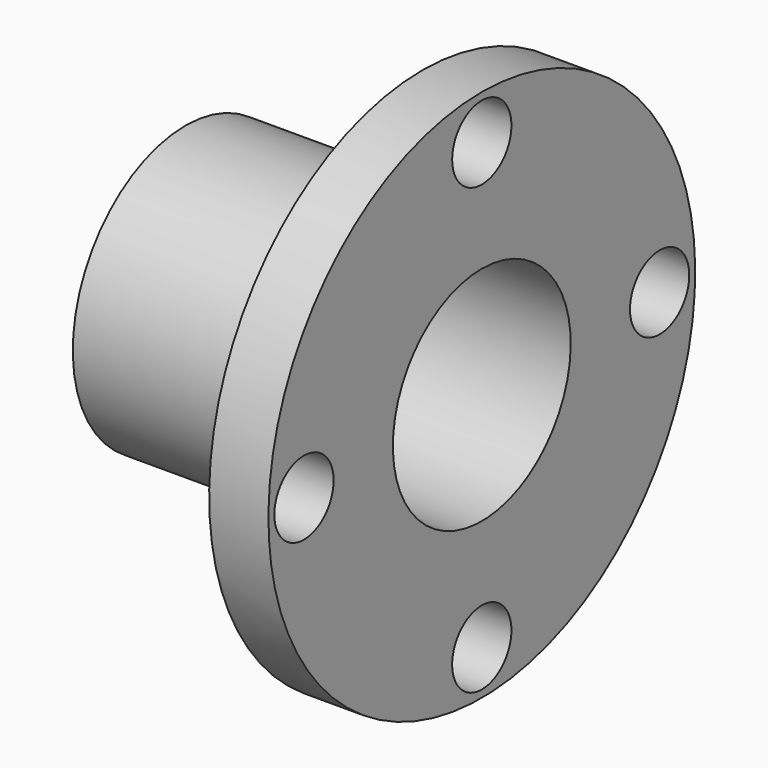
from build123d import *

# Parameters (mm, degrees)
F2_R            = 12.5
F3_DEPTH        = 25
F3_COPIES_COUNT = 4


# Not quite as in the source:
# - a pattern or mirror of a feature is missing from the dataset's text; its kind, count and spacing are read off the source's solid


with BuildPart() as f1:
    # F0 (on Front) → F1 (revolve)
    with BuildSketch(Plane.XZ):
        Polygon((-100, 37.5), (0, 37.5), (0, 90), (-20, 90), (-20, 47.5), (-100, 47.5), align=None)
    revolve(axis=Axis((-58.4905732034, 0, 0), (-1, 0, 0)))

    # F2 (on face) → F3 (cut)
    with BuildSketch(Plane(origin=(-20, 0, 0), x_dir=(0, -1, 0), z_dir=(-1, 0, 0))):
        with Locations((0, 75)):
            Circle(F2_R)
    f3 = extrude(amount=-F3_DEPTH, mode=Mode.SUBTRACT)

    # F3_copies: F3 ×4 about axis
    f3_copies_axis = Axis((0, 0, 0), (1, 0, 0))
    for i in range(1, F3_COPIES_COUNT):
        add(f3.rotate(f3_copies_axis, i * 360 / F3_COPIES_COUNT), mode=Mode.SUBTRACT)


solid = f1.part
